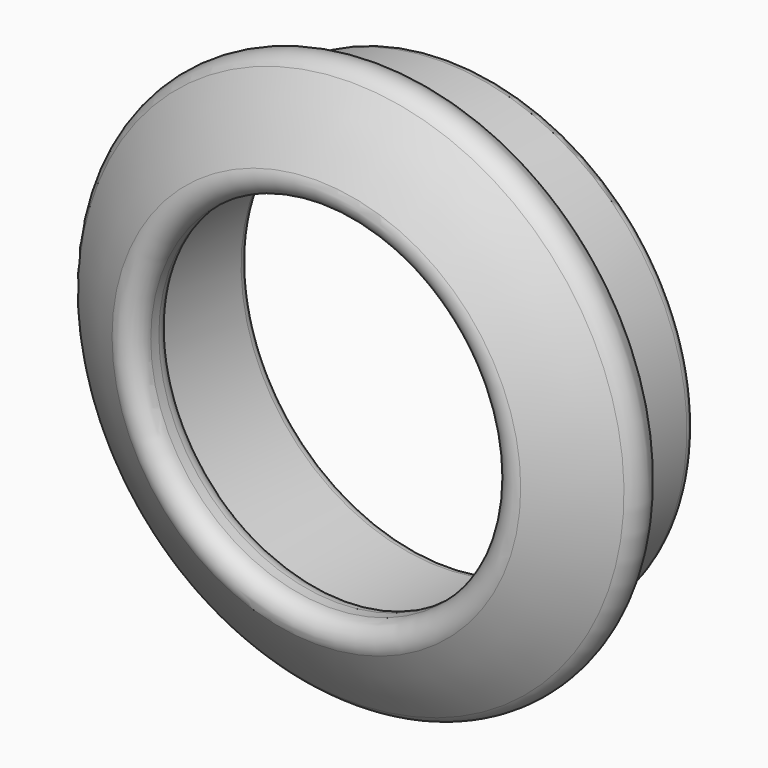
from build123d import *


# Not quite as in the source:
# - ends of sketch curves that miss each other by under 0.0002 mm in the source are joined


with BuildPart() as f1:
    # F0 (on Right) → F1 (revolve)
    with BuildSketch(Plane.YZ):
        with BuildLine():
            ThreePointArc((-2.2311331873, 4.5833333333), (-2.2171860627, 4.1918334001), (-1.8756210372, 4))
            Line((-1.8756210372, 4), (-1.6499533041, 4))
            ThreePointArc((-1.6499533041, 4), (-1.4436690548, 4.0572948666), (-1.2964799482, 4.2127659576))
            ThreePointArc((-1.2964799482, 4.2127659576), (-1.2183286985, 4.3571076069), (-1.1375580754, 4.5))
            ThreePointArc((-1.1375580754, 4.5), (-0.8191484877, 5.0112004142), (-0.4672628718, 5.4999611351))
            ThreePointArc((-0.4672628718, 5.4999611351), (-0.4648905545, 5.5030325568), (-0.462516913, 5.5061029552))
            ThreePointArc((-0.462516913, 5.5061029552), (-0.3625691061, 5.8792370625), (-0.5583476801, 6.2122376272))
            ThreePointArc((-0.558347675, 6.2122376234), (-0.925266822, 6.3074557819), (-1.2535377384, 6.1178921683))
            ThreePointArc((-1.2535377384, 6.1178921683), (-1.7773095132, 5.3728930777), (-2.2311331873, 4.5833333333))
        make_face()
        with BuildLine():
            ThreePointArc((-0.4672628718, 5.4999611351), (-0.8191484877, 5.0112004142), (-1.1375580754, 4.5))
            Line((-1.1375580754, 4.5), (1.2826867876, 4.5))
            ThreePointArc((1.2826867876, 4.5), (1.4594634829, 4.5732233047), (1.5326867876, 4.75))
            Line((1.5326867876, 4.75), (1.5326867876, 5.25))
            ThreePointArc((1.5326867876, 5.25), (1.4594634829, 5.4267766953), (1.2826867876, 5.5))
            Line((1.2826867876, 5.5), (-0.4672628718, 5.4999611351))
        make_face()
    revolve(axis=Axis((0, -2.6926244609, 0), (0, -1, 0)))


solid = f1.part
